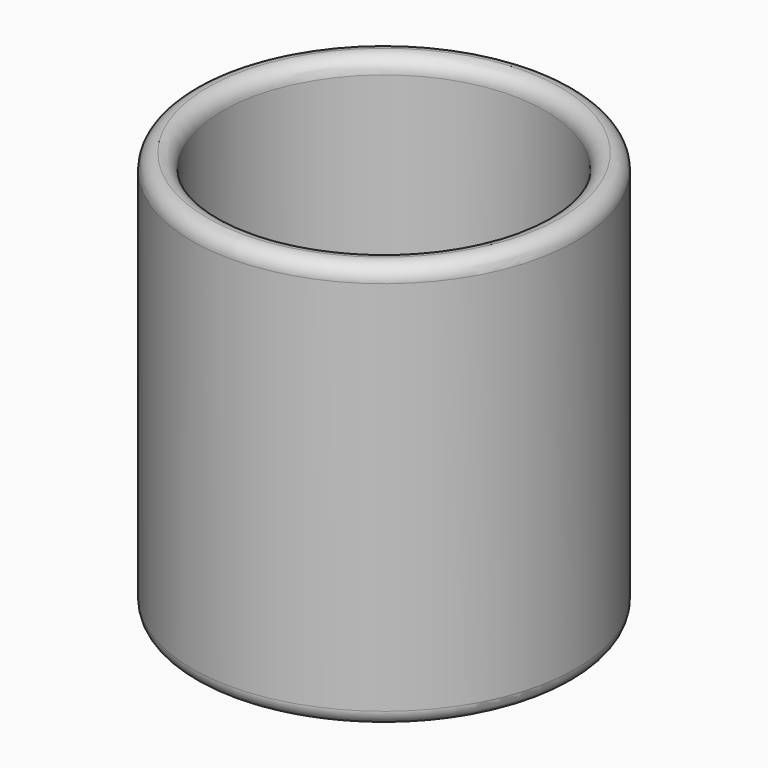
from build123d import *

# Parameters (mm, degrees)
F0_R     = 25
F1_DEPTH = 3
F2_R     = 25
F2_R_2   = 21
F3_DEPTH = 50
F4_R     = 1.99999
F5_R     = 2


# Not quite as in the source:
# - a fillet or chamfer is up to 0.001 mm smaller than in the source, because OpenCascade refuses the exact size


with BuildPart() as f1:
    # F0 (on Top) → F1 (new body)
    with BuildSketch(Plane.XY):
        Circle(F0_R)
    extrude(amount=F1_DEPTH)

    # F2 (on face) → F3 (join)
    with BuildSketch(Plane.XY.offset(3)):
        Circle(F2_R)
        Circle(F2_R_2, mode=Mode.SUBTRACT)
    extrude(amount=F3_DEPTH)

    # F4 (radius 2 in the source; OpenCascade refuses exactly that, so slightly less here)
    f4_edges = [f1.edges().sort_by_distance(p)[0] for p in [
        (-25, 0, 53),
        (-21, 0, 53),
        (-21, 0, 3),
    ]]
    fillet(f4_edges, radius=F4_R)

    # F5
    f5_edges = [f1.edges().sort_by_distance(p)[0] for p in [
        (-25, 0, 0),
    ]]
    fillet(f5_edges, radius=F5_R)


solid = f1.part
